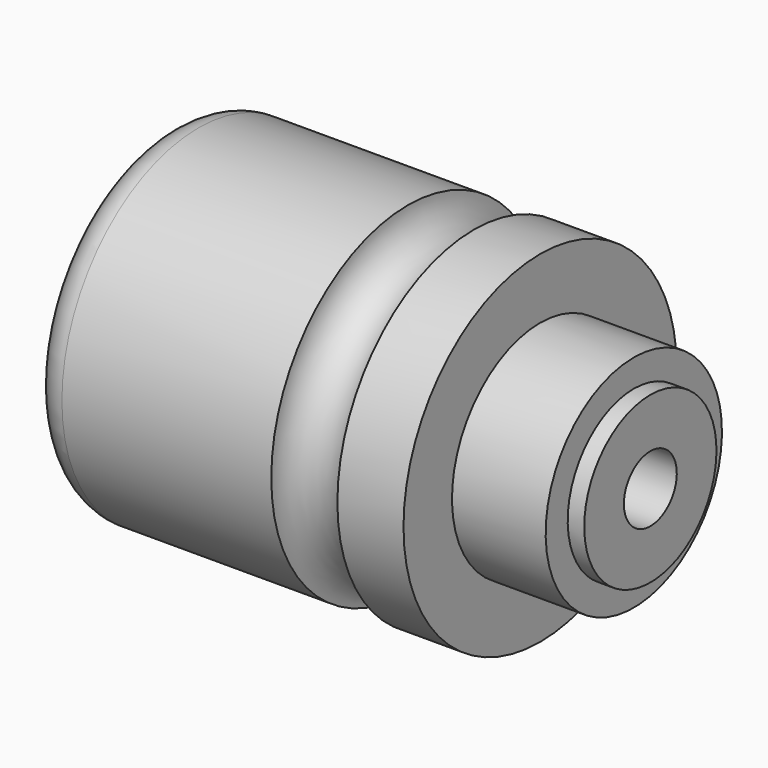
from build123d import *

# Parameters (mm, degrees)
F4_R = 5.99999


# Not quite as in the source:
# - a fillet or chamfer is up to 0.001 mm smaller than in the source, because OpenCascade refuses the exact size


with BuildPart() as f1:
    # F0 (on Front) → F1 (revolve)
    with BuildSketch(Plane.XZ):
        with BuildLine():
            Line((0, 31), (0, 0))
            Line((0, 0), (88, 0))
            Line((88, 0), (88, 15))
            Line((88, 15), (85, 15))
            Line((85, 15), (85, 20))
            Line((85, 20), (68, 20))
            Line((68, 20), (68, 31))
            Line((68, 31), (56, 31))
            ThreePointArc((56, 31), (50, 25), (44, 31))
            Line((44, 31), (0, 31))
        make_face()
    revolve(axis=Axis((63.3454471827, 0, 0), (1, 0, 0)))

    # F2 (on Front) → F3 (revolve, cut)
    with BuildSketch(Plane.XZ):
        Polygon((0, 25), (0, 0), (88, 0), (88, 6), (30, 6), (30, 16), (22, 16), (22, 20.5), (12, 20.5), (12, 12.5), (9, 12.5), (9, 16), (1.5, 16), (1.5, 25), align=None)
    revolve(axis=Axis((-10.8097042758, 0, 0), (-1, 0, 0)), mode=Mode.SUBTRACT)

    # F4 (radius 6 in the source; OpenCascade refuses exactly that, so slightly less here)
    f4_edges = [f1.edges().sort_by_distance(p)[0] for p in [
        (0, 0, -31),
    ]]
    fillet(f4_edges, radius=F4_R)


solid = f1.part
